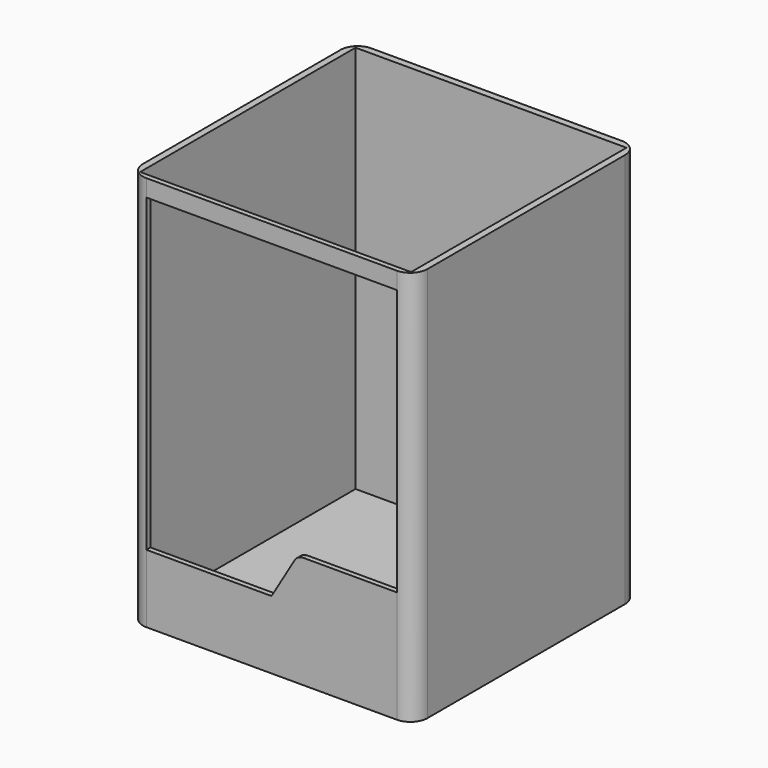
from build123d import *

# Parameters (mm, degrees)
F0_W     = 83.5
F0_H     = 82.5
F1_DEPTH = 116
F3_DEPTH = 25
F4_R     = 3
F5_DEPTH = 2
F6_R     = 4.99999


# Not quite as in the source:
# - a fillet or chamfer is up to 0.001 mm smaller than in the source, because OpenCascade refuses the exact size


with BuildPart() as f1:
    # F0 (on Top) → F1 (new body)
    with BuildSketch(Plane.XY):
        with Locations((-41.75, 41.25)):
            Rectangle(F0_W, F0_H)
        Polygon((-2, 1.5), (-43.8047535717, 1.5), (-81.5, 1.5), (-81.5, 41.25), (-81.5, 80.5), (-41.75, 80.5), (-2, 80.5), (-2, 41.25), align=None, mode=Mode.SUBTRACT)
    extrude(amount=F1_DEPTH)

    # F2 (on Front) → F3 (cut)
    with BuildSketch(Plane.XZ):
        Polygon((-5, 111), (-78.5, 111), (-78.5, 20), (-41.75, 20), (-34.1152064502, 32.9003408551), (-5, 32.9003408551), align=None)
    extrude(amount=-F3_DEPTH, mode=Mode.SUBTRACT)

    # F4
    f4_edges = [f1.edges().sort_by_distance(p)[0] for p in [
        (-34.115206, 0.75, 32.900341),
    ]]
    fillet(f4_edges, radius=F4_R)

    # F0 (on Top) → F5 (join)
    with BuildSketch(Plane.XY):
        Polygon((-81.5, 1.5), (-43.8047535717, 1.5), (-2, 1.5), (-2, 41.25), (-2, 80.5), (-41.75, 80.5), (-81.5, 80.5), (-81.5, 41.25), align=None)
    extrude(amount=F5_DEPTH)

    # F6 (radius 5 in the source; OpenCascade refuses exactly that, so slightly less here)
    f6_edges = [f1.edges().sort_by_distance(p)[0] for p in [
        (-83.5, 0, 58),
        (0, 0, 58),
        (0, 82.5, 58),
        (-83.5, 82.5, 58),
    ]]
    fillet(f6_edges, radius=F6_R)


solid = f1.part
